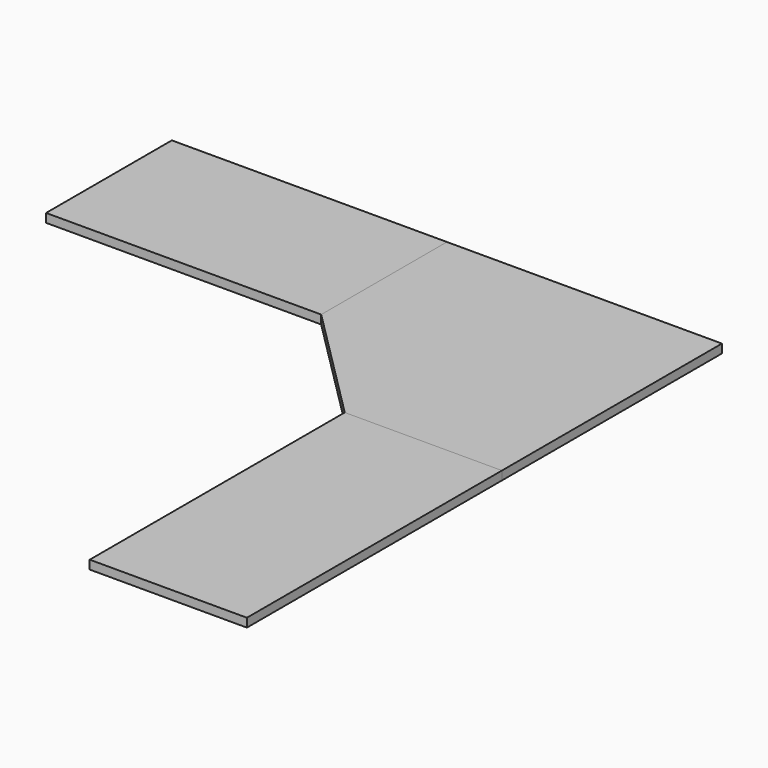
from build123d import *

# Parameters (mm, degrees)
F2_W     = 800.2447458586
F2_H     = 457.2
F4_DEPTH = 25.4
F5_DEPTH = 25.4
F3_W     = 457.2
F3_H     = 927.2447458586
F6_DEPTH = 25.4


with BuildPart() as f4:
    # F2 (on face) → F4 (new body)
    with BuildSketch(Plane.XY):
        with Locations((-1200.0776270707, -228.6)):
            Rectangle(F2_W, F2_H)
    extrude(amount=-F4_DEPTH)


with BuildPart() as f5:
    # F3 (on face) → F5 (new body)
    with BuildSketch(Plane.XY):
        Polygon((-457.2, -799.9552541414), (0, -799.9552541414), (0, 0), (-799.9552541414, 0), (-799.9552541414, -457.2), align=None)
    extrude(amount=-F5_DEPTH)


with BuildPart() as f6:
    # F3 (on face) → F6 (new body)
    with BuildSketch(Plane.XY):
        with Locations((-228.6, -1263.5776270707)):
            Rectangle(F3_W, F3_H)
    extrude(amount=-F6_DEPTH)


solid = Compound([f4.part, f5.part, f6.part])
